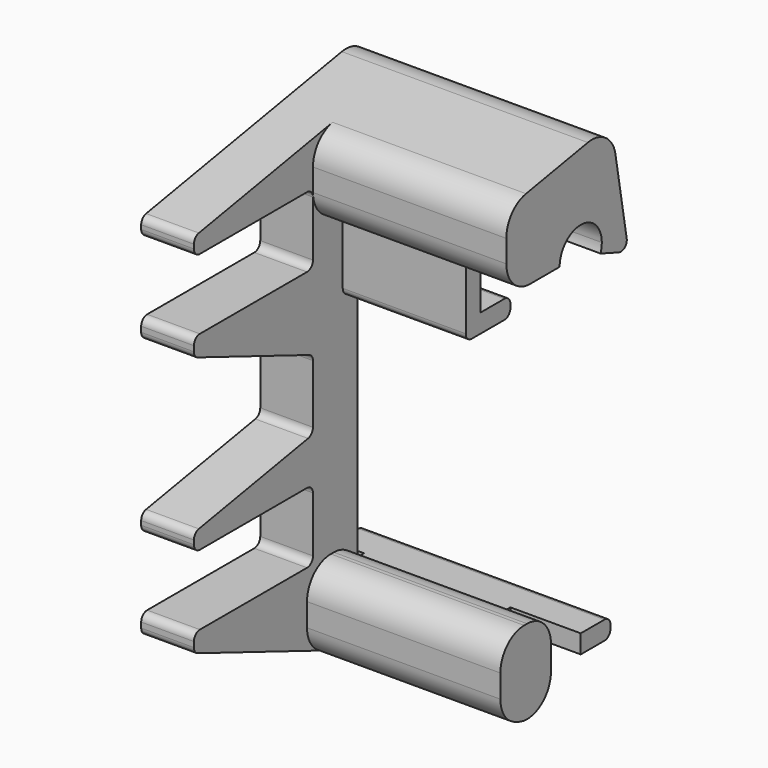
from build123d import *

# Parameters (mm, degrees)
F1_DEPTH       = 42
F2_R           = 5.08
F3_R           = 1.27
F4_W           = 25
F4_H           = 3.175
F5_DEPTH       = 12.7
F7_DEPTH       = 33
F8_T1_DEPTH    = 45.7
F8_T3_DEPTH    = 43.656565316
F8_T5_DEPTH    = 41.6709689227
F9_W           = 6.35
F9_H           = 3.175
F10_DEPTH      = 12
F10_DEPTH_BACK = 30
F12_DEPTH      = 21
F12_DEPTH_BACK = 4
F13_R          = 1.27


# Not quite as in the source:
# - a fillet or chamfer that OpenCascade refuses, or shapes differently, is made with other operations: its cross-section is extruded or revolved along the edge and cut away or added


with BuildPart() as f1:
    # F0 (on Right) → F1 (new body)
    with BuildSketch(Plane.YZ):
        with BuildLine():
            Line((0, 0), (0, 67.502))
            Line((0, 67.502), (1.85, 67.502))
            ThreePointArc((1.85, 67.502), (6.35, 72.002), (10.85, 67.502))
            ThreePointArc((10.85, 67.502), (10.7816348886, 66.7205832005), (10.5786167935, 65.962909355))
            Line((10.5786167935, 65.962909355), (16.5456649355, 63.7910814449))
            Line((16.5456649355, 63.7910814449), (12.8715844298, 84.6278274207))
            Line((12.8715844298, 84.6278274207), (-34.925, 76.2))
            Line((-34.925, 76.2), (-34.925, 73.152))
            Line((-34.925, 73.152), (-9.525, 73.152))
            Line((-9.525, 73.152), (-9.525, 61.152))
            Line((-9.525, 61.152), (-34.925, 61.152))
            Line((-34.925, 61.152), (-34.925, 58.104))
            Line((-34.925, 58.104), (-9.525, 48.1738181818))
            Line((-9.525, 48.1738181818), (-9.525, 36.22870531))
            Line((-9.525, 36.22870531), (-34.925, 31.75))
            Line((-34.925, 31.75), (-34.925, 28.702))
            Line((-34.925, 28.702), (-9.525, 28.702))
            Line((-9.525, 28.702), (-9.525, 16.702))
            Line((-9.525, 16.702), (-34.925, 16.702))
            Line((-34.925, 16.702), (-34.925, 13.654))
            Line((-34.925, 13.654), (0, 0))
        make_face()
    extrude(amount=F1_DEPTH)

    # F2
    f2_edges = [f1.edges().sort_by_distance(p)[0] for p in [
        (21, 12.871584, 84.627827),
        (21, 0, 0),
    ]]
    fillet(f2_edges, radius=F2_R)

    # F3
    f3_edges = [f1.edges().sort_by_distance(p)[0] for p in [
        (21, 16.545665, 63.791081),
        (21, -9.525, 28.702),
        (21, -9.525, 48.173818),
        (21, -9.525, 73.152),
        (21, -9.525, 61.152),
        (21, -9.525, 16.702),
        (21, -34.925, 16.702),
        (21, -34.925, 13.654),
        (21, -34.925, 28.702),
        (21, -34.925, 61.152),
        (21, -34.925, 58.104),
        (21, -34.925, 31.75),
        (21, -34.925, 73.152),
        (21, -34.925, 76.2),
        (21, -9.525, 36.228705),
    ]]
    fillet(f3_edges, radius=F3_R)

    # F4 (on face) → F5 (join)
    with BuildSketch(Plane(origin=(0, 0, 0), x_dir=(-1, 0, 0), z_dir=(0, 1, 0))):
        with Locations((-17.5, 9.0279602963)):
            Rectangle(F4_W, F4_H)
    extrude(amount=F5_DEPTH)

    # F6 (on face) → F7 (cut)
    with BuildSketch(Plane.YZ.offset(42)):
        Polygon((0, 16.702), (0, 67.502), (-9.525, 67.502), (-9.525, 80.67870531), (-34.925, 80.67870531), (-34.925, 4.2203272727), (-10.795, 4.2203272727), (-10.795, 16.702), align=None)
    extrude(amount=-F7_DEPTH, mode=Mode.SUBTRACT)

    # F8: fillet of radius 5.08 on 5 edges, made by hand

    # F8_s2 → F8_t1 (cut)
    with BuildSketch(Plane.YZ.offset(9)):
        with BuildLine():
            ThreePointArc((-4.445, 67.502), (-8.0371024484, 68.9898975516), (-9.525, 72.582))
            Line((-9.525, 72.582), (-9.525, 67.502))
            Line((-9.525, 67.502), (-4.445, 67.502))
        make_face()
        with BuildLine():
            ThreePointArc((-5.715, 16.702), (-9.3071024484, 15.2141024484), (-10.795, 11.622))
            Line((-10.795, 11.622), (-10.795, 16.702))
            Line((-10.795, 16.702), (-5.715, 16.702))
        make_face()
        with BuildLine():
            ThreePointArc((-5.08, 16.702), (-1.4878975516, 15.2141024484), (0, 11.622))
            Line((0, 11.622), (0, 16.702))
            Line((0, 16.702), (-5.08, 16.702))
        make_face()
    extrude(amount=F8_T1_DEPTH, mode=Mode.SUBTRACT)

    # F8_s4 → F8_t3 (cut)
    with BuildSketch(Plane.YZ.offset(9)):
        with BuildLine():
            ThreePointArc((-5.3271327425, 81.4189025689), (-8.336505771, 79.6814402408), (-9.525, 76.4160791836))
            Line((-9.525, 76.4160791836), (-9.525, 80.67870531))
            Line((-9.525, 80.67870531), (-5.3271327425, 81.4189025689))
        make_face()
    extrude(amount=F8_T3_DEPTH, mode=Mode.SUBTRACT)

    # F8_s6 → F8_t5 (cut)
    with BuildSketch(Plane.YZ.offset(9)):
        with BuildLine():
            ThreePointArc((-10.795, 7.6887148418), (-9.9104077053, 4.8242857213), (-7.5647030762, 2.9574361003))
            Line((-7.5647030762, 2.9574361003), (-10.795, 4.2203272727))
            Line((-10.795, 4.2203272727), (-10.795, 7.6887148418))
        make_face()
    extrude(amount=F8_T5_DEPTH, mode=Mode.SUBTRACT)

    # F9 (on face) → F10 (join, two sides)
    with BuildSketch(Plane.YZ.offset(30)) as f10_sk:
        with Locations((9.525, 9.0279602963)):
            Rectangle(F9_W, F9_H)
    extrude(amount=F10_DEPTH)
    extrude(f10_sk.sketch, amount=-F10_DEPTH_BACK)

    # F11 (on face) → F12 (join, two sides)
    with BuildSketch(Plane.YZ.offset(9)) as f12_sk:
        Polygon((0, 57.502), (0, 67.502), (-3.175, 67.502), (-3.175, 54.327), (6.35, 54.327), (6.35, 57.502), align=None)
    extrude(amount=F12_DEPTH)
    extrude(f12_sk.sketch, amount=-F12_DEPTH_BACK)

    # F13
    f13_edges = [f1.edges().sort_by_distance(p)[0] for p in [
        (21, 12.7, 10.61546),
        (21, 12.7, 7.44046),
        (17.5, 6.35, 57.502),
        (17.5, 6.35, 54.327),
        (19.5, -3.175, 54.327),
    ]]
    fillet(f13_edges, radius=F13_R)


solid = f1.part
